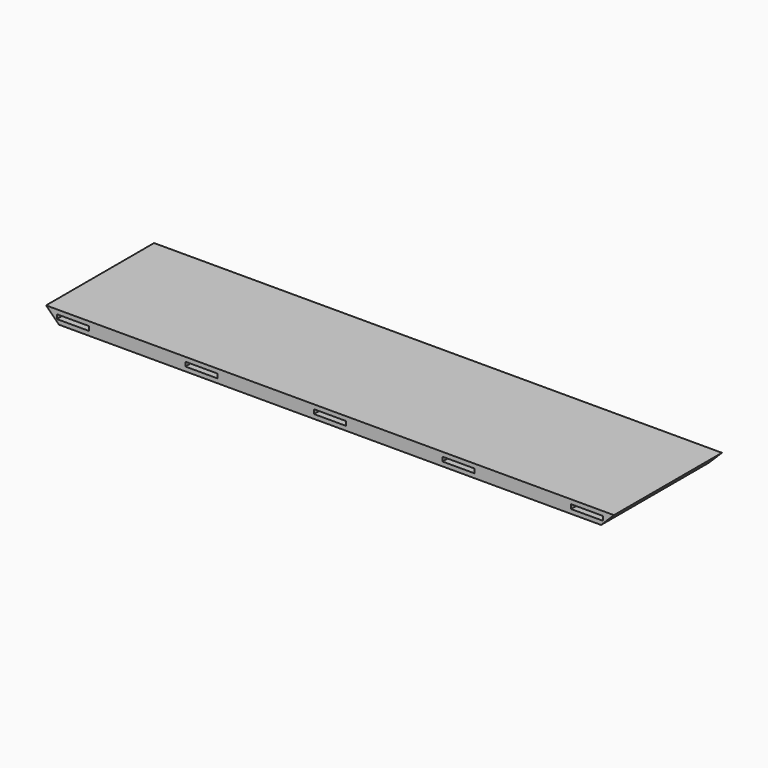
from build123d import *

# Parameters (mm, degrees)
F1_W     = 1200
F1_H     = 210
F2_DEPTH = 10
F3_W     = 50
F3_H     = 6.6666666667
F4_DEPTH = 15
F6_DEPTH = 210.001


# Not quite as in the source:
# - a pattern or mirror of a feature is missing from the dataset's text; its kind, count and spacing are read off the source's solid


with BuildPart() as f2:
    # F1 (on Top) → F2 (new body, symmetric)
    with BuildSketch(Plane.XY):
        Rectangle(F1_W, F1_H)
    extrude(amount=F2_DEPTH, both=True)

    # F3 (on face) → F4 (cut)
    with BuildSketch(Plane.XZ.offset(105)):
        Rectangle(F3_W, F3_H)
        with Locations((200, 0)):
            Rectangle(F3_W, F3_H)
        with Locations((400, 0)):
            Rectangle(F3_W, F3_H)
        with Locations((-200, 0)):
            Rectangle(F3_W, F3_H)
        with Locations((-400, 0)):
            Rectangle(F3_W, F3_H)
    f4 = extrude(amount=-F4_DEPTH, mode=Mode.SUBTRACT)

    # F4_copies: F4 across plane
    add(f4.mirror(Plane.ZX), mode=Mode.SUBTRACT)

    # F5 (on face) → F6 (cut, through all)
    with BuildSketch(Plane.XZ.offset(105)):
        Polygon((-421.7155, -10), (-441.7155, 10), (-600, 10), (-600, -10), align=None)
        Polygon((600, -10), (600, 10), (441.7155, 10), (421.7155, -10), align=None)
    extrude(amount=-F6_DEPTH, mode=Mode.SUBTRACT)


solid = f2.part
